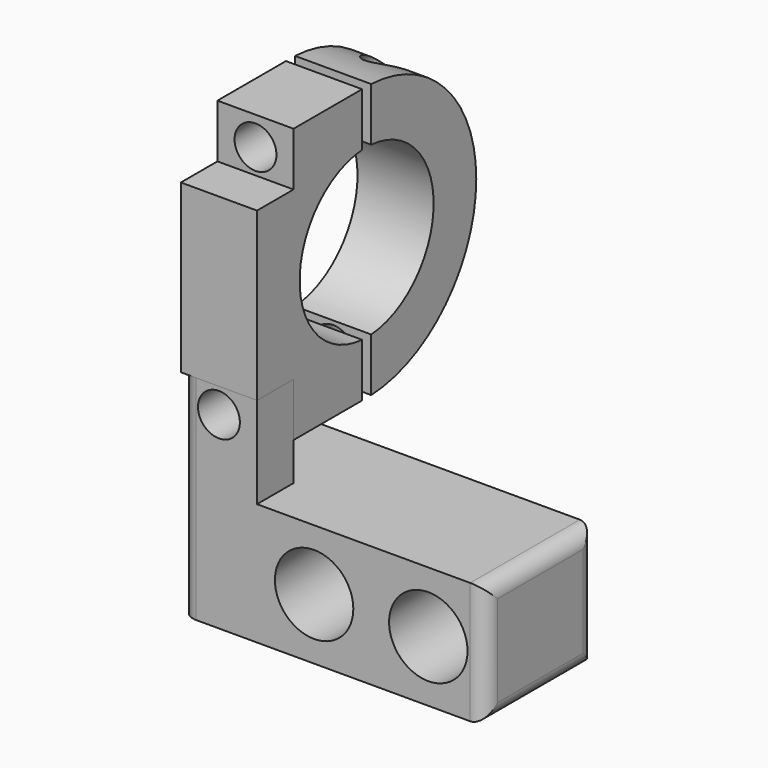
from build123d import *

# Parameters (mm, degrees)
F1_DEPTH      = 5
F2_R          = 2.75
F3_DEPTH      = 12.5
F4_W          = 10
F4_H          = 4.9744020338
F4_H_2        = 7.0255979662
F4_R          = 2.75
F5_DEPTH      = 6
F6_DEPTH      = 6
F6_DEPTH_BACK = 12
F7_R          = 5.15
F8_DEPTH      = 18
F9_DEPTH      = 18
F11_R         = 2


# Not quite as in the source:
# - the program builds the solid bodies; features that only make, move or delete a surface that nothing else refers to are left out


with BuildPart() as f1:
    # F0 (on Right) → F1 (new body, symmetric)
    with BuildSketch(Plane.YZ):
        with BuildLine():
            ThreePointArc((-0.75, -10.9744020338), (-11, 0), (-0.75, 10.9744020338))
            Line((-0.75, 10.9744020338), (-0.75, 18))
            Line((-0.75, 18), (-12, 18))
            Line((-12, 18), (-12, 10.9744020338))
            Line((-12, 10.9744020338), (-18, 10.9744020338))
            Line((-18, 10.9744020338), (-18, -10.9744020338))
            Line((-18, -10.9744020338), (-12, -10.9744020338))
            Line((-12, -10.9744020338), (-12, -18))
            Line((-12, -18), (-0.75, -18))
            Line((-0.75, -18), (-0.75, -10.9744020338))
        make_face()
    extrude(amount=F1_DEPTH, both=True)


with BuildPart() as f1b:
    # F0 (on Right) → F1, piece 2 (new body, symmetric)
    with BuildSketch(Plane.YZ):
        with BuildLine():
            Line((0.75, -10.9744020338), (0.75, -17.9843682124))
            ThreePointArc((0.75, -17.9843682124), (18, 0), (0.75, 17.9843682124))
            Line((0.75, 17.9843682124), (0.75, 10.9744020338))
            ThreePointArc((0.75, 10.9744020338), (11, 0), (0.75, -10.9744020338))
        make_face()
    extrude(amount=F1_DEPTH, both=True)


with BuildPart() as f3_tool:
    # F2 (on Front) → F3 (new body, symmetric)
    with BuildSketch(Plane.XZ):
        with Locations((0, 14.25)):
            Circle(F2_R)
        with Locations((0, -14.25)):
            Circle(F2_R)
    extrude(amount=F3_DEPTH, both=True)


with BuildPart() as f1_1:
    add(f1.part)

    # F3: cut by f3_tool
    add(f3_tool.part, mode=Mode.SUBTRACT)


with BuildPart() as f1b_1:
    add(f1b.part)

    # F3: cut by f3_tool
    add(f3_tool.part, mode=Mode.SUBTRACT)


with BuildPart() as f5:
    # F4 (on face) → F5 (new body, through all)
    with BuildSketch(Plane.XZ.offset(12)):
        with Locations((0, -20.4872010169)):
            Rectangle(F4_W, F4_H)
        with Locations((0, -14.4872010169)):
            Rectangle(F4_W, F4_H_2)
        with Locations((0, -14.25)):
            Circle(F4_R, mode=Mode.SUBTRACT)
    extrude(amount=F5_DEPTH)

    # F4 (on face) → F6 (join, two sides)
    with BuildSketch(Plane.XZ.offset(12)) as f6_sk:
        Polygon((5, -22.9744020338), (-5, -22.9744020338), (-5, -38.9744020338), (35, -38.9744020338), (35, -22.9744020338), align=None)
    extrude(amount=F6_DEPTH)
    extrude(f6_sk.sketch, amount=-F6_DEPTH_BACK)

    # F7 (on face) → F8 (cut, through all)
    with BuildSketch(Plane.XZ.offset(18)):
        with Locations((12.5, -30.9744020338)):
            Circle(F7_R)
    extrude(amount=-F8_DEPTH, mode=Mode.SUBTRACT)

    # F7 (on face) → F9 (cut, through all)
    with BuildSketch(Plane.XZ.offset(18)):
        with Locations((27.5, -30.9744020338)):
            Circle(F7_R)
    extrude(amount=-F9_DEPTH, mode=Mode.SUBTRACT)

    # F11
    f11_edges = [f5.edges().sort_by_distance(p)[0] for p in [
        (35, -18, -30.974402),
        (35, 0, -30.974402),
        (35, -9, -38.974402),
        (35, -9, -22.974402),
        (-5, -18, -24.974402),
    ]]
    fillet(f11_edges, radius=F11_R)


solid = Compound([f1_1.part, f1b_1.part, f5.part])
